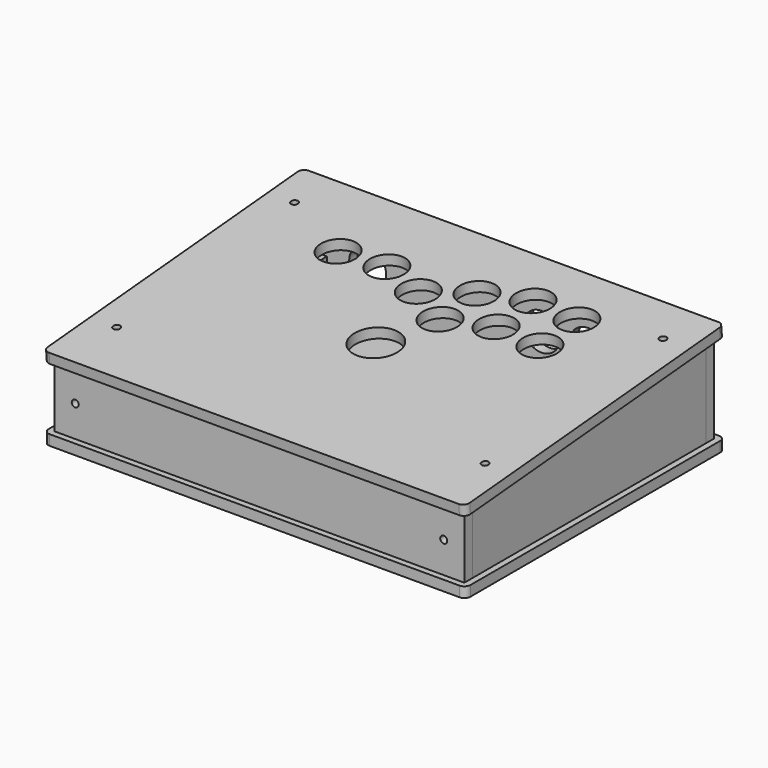
from build123d import *

# Parameters (mm, degrees)
F0_W      = 12.5984
F0_H      = 4.572
F0_W_2    = 3.048
F0_W_3    = 4.572
F0_H_2    = 12.5984
F0_H_3    = 3.048
F0_H_4    = 2.286
F0_W_4    = 2.286
F1_DEPTH  = 6.7056
F2_DEPTH  = 6.7056
F4_DEPTH  = 6.7056
F7_DEPTH  = 266.7
F8_R      = 2.286
F10_DEPTH = 6.7056
F9_R      = 2.286
F11_DEPTH = 6.7056
F12_W     = 266.7
F12_H     = 203.9761909888
F12_R     = 2.286
F12_R_2   = 15
F12_R_3   = 12
F12_W_2   = 6.7056
F12_H_2   = 190.5137623835
F13_DEPTH = 6.7056
F14_W     = 266.7
F14_H     = 203.2
F14_R     = 2.286
F14_W_2   = 6.7056
F14_H_2   = 189.7888
F15_DEPTH = 6.7056
F16_R     = 12
F16_R_2   = 1.6
F17_DEPTH = 6.7056


# Not quite as in the source:
# - a feature names something its author has since deleted; it is built from what else it names


with BuildPart() as f1:
    # F0 (on Right) → F1 (new body)
    with BuildSketch(Plane.YZ):
        Polygon((-94.8944, -2.286), (-94.8944, -20.32), (-69.4944, -20.32), (-69.4944, -7.7216), (-71.7804, -7.7216), (-71.7804, -4.6736), (-69.4944, -4.6736), (-69.4944, -1.6256), (-64.9224, -1.6256), (-64.9224, -4.6736), (-62.6364, -4.6736), (-62.6364, -7.7216), (-64.9224, -7.7216), (-64.9224, -20.32), (75.0824, -20.32), (75.0824, -7.7216), (72.7964, -7.7216), (72.7964, -4.6736), (75.0824, -4.6736), (75.0824, -1.6256), (79.6544, -1.6256), (79.6544, -4.6736), (81.9404, -4.6736), (81.9404, -7.7216), (79.6544, -7.7216), (79.6544, -20.32), (94.8944, -20.32), (94.8944, 6.6028482142), (82.296, 6.6028482142), (82.296, 4.3168482142), (79.248, 4.3168482142), (79.248, 6.6028482142), (76.2, 6.6028482142), (76.2, 11.1748482142), (79.248, 11.1748482142), (79.248, 13.4608482142), (82.296, 13.4608482142), (82.296, 11.1748482142), (94.8944, 11.1748482142), (94.8944, 37.5110324463), (79.7123928011, 36.1827789269), (80.8104157105, 23.6323196424), (83.0877167904, 23.8315576703), (83.3533674942, 20.7951562306), (81.0760664144, 20.5959182026), (81.3417171183, 17.5595167628), (76.7871149586, 17.161040707), (76.5214642547, 20.1974421468), (74.2441631749, 19.9982041189), (73.978512471, 23.0346055587), (76.2558135508, 23.2338435866), (75.1577906414, 35.784302871), (-65.0364525088, 23.5188959038), (-63.9384295994, 10.9684366193), (-61.6611285195, 11.1676746473), (-61.3954778156, 8.1312732075), (-63.6727788955, 7.9320351795), (-63.4071281916, 4.8956337398), (-67.9617303512, 4.4971576839), (-68.2273810551, 7.5335591237), (-70.504682135, 7.3343210958), (-70.7703328389, 10.3707225356), (-68.493031759, 10.5699605635), (-69.5910546685, 23.1204198479), (-94.8944, 20.9066639821), (-94.8944, 2.286), (-82.296, 2.286), (-82.296, 4.572), (-79.248, 4.572), (-79.248, 2.286), (-76.2, 2.286), (-76.2, -2.286), (-79.248, -2.286), (-79.248, -4.572), (-82.296, -4.572), (-82.296, -2.286), align=None)
        Polygon((79.7123928011, 36.1827789269), (75.1577906414, 35.784302871), (76.2558135508, 23.2338435866), (80.8104157105, 23.6323196424), align=None)
        Polygon((80.8104157105, 23.6323196424), (76.2558135508, 23.2338435866), (76.5214642547, 20.1974421468), (81.0760664144, 20.5959182026), align=None)
        Polygon((81.0760664144, 20.5959182026), (76.5214642547, 20.1974421468), (76.7871149586, 17.161040707), (81.3417171183, 17.5595167628), align=None)
        Polygon((-65.0364525088, 23.5188959038), (-69.5910546685, 23.1204198479), (-68.493031759, 10.5699605635), (-63.9384295994, 10.9684366193), align=None)
        Polygon((-63.9384295994, 10.9684366193), (-68.493031759, 10.5699605635), (-68.2273810551, 7.5335591237), (-63.6727788955, 7.9320351795), align=None)
        Polygon((-63.6727788955, 7.9320351795), (-68.2273810551, 7.5335591237), (-67.9617303512, 4.4971576839), (-63.4071281916, 4.8956337398), align=None)
        with Locations((-88.5952, 0)):
            Rectangle(F0_W, F0_H)
        with Locations((-80.772, 0)):
            Rectangle(F0_W_2, F0_H)
        with Locations((-77.724, 0)):
            Rectangle(F0_W_2, F0_H)
        with Locations((-67.2084, -14.0208)):
            Rectangle(F0_W_3, F0_H_2)
        with Locations((-67.2084, -6.1976)):
            Rectangle(F0_W_3, F0_H_3)
        with Locations((-67.2084, -3.1496)):
            Rectangle(F0_W_3, F0_H_3)
        with Locations((77.3684, -14.0208)):
            Rectangle(F0_W_3, F0_H_2)
        with Locations((77.3684, -6.1976)):
            Rectangle(F0_W_3, F0_H_3)
        with Locations((77.3684, -3.1496)):
            Rectangle(F0_W_3, F0_H_3)
        with Locations((88.5952, 8.8888482142)):
            Rectangle(F0_W, F0_H)
        with Locations((80.772, 8.8888482142)):
            Rectangle(F0_W_2, F0_H)
        with Locations((77.724, 8.8888482142)):
            Rectangle(F0_W_2, F0_H)
        Polygon((76.5214642547, 20.1974421468), (76.2558135508, 23.2338435866), (73.978512471, 23.0346055587), (74.2441631749, 19.9982041189), align=None)
        Polygon((83.0877167904, 23.8315576703), (80.8104157105, 23.6323196424), (81.0760664144, 20.5959182026), (83.3533674942, 20.7951562306), align=None)
        with Locations((80.772, 5.4598482142)):
            Rectangle(F0_W_2, F0_H_4)
        with Locations((80.772, 12.3178482142)):
            Rectangle(F0_W_2, F0_H_4)
        with Locations((80.7974, -6.1976)):
            Rectangle(F0_W_4, F0_H_3)
        with Locations((73.9394, -6.1976)):
            Rectangle(F0_W_4, F0_H_3)
        with Locations((-63.7794, -6.1976)):
            Rectangle(F0_W_4, F0_H_3)
        with Locations((-70.6374, -6.1976)):
            Rectangle(F0_W_4, F0_H_3)
        with Locations((-80.772, -3.429)):
            Rectangle(F0_W_2, F0_H_4)
        with Locations((-80.772, 3.429)):
            Rectangle(F0_W_2, F0_H_4)
        Polygon((-68.2273810551, 7.5335591237), (-68.493031759, 10.5699605635), (-70.7703328389, 10.3707225356), (-70.504682135, 7.3343210958), align=None)
        Polygon((-61.6611285195, 11.1676746473), (-63.9384295994, 10.9684366193), (-63.6727788955, 7.9320351795), (-61.3954778156, 8.1312732075), align=None)
    extrude(amount=-F1_DEPTH)


with BuildPart() as f2:
    # F0 (on Right) → F2 (new body)
    with BuildSketch(Plane.YZ):
        Polygon((-94.8944, -2.286), (-94.8944, -20.32), (-69.4944, -20.32), (-69.4944, -7.7216), (-71.7804, -7.7216), (-71.7804, -4.6736), (-69.4944, -4.6736), (-69.4944, -1.6256), (-64.9224, -1.6256), (-64.9224, -4.6736), (-62.6364, -4.6736), (-62.6364, -7.7216), (-64.9224, -7.7216), (-64.9224, -20.32), (75.0824, -20.32), (75.0824, -7.7216), (72.7964, -7.7216), (72.7964, -4.6736), (75.0824, -4.6736), (75.0824, -1.6256), (79.6544, -1.6256), (79.6544, -4.6736), (81.9404, -4.6736), (81.9404, -7.7216), (79.6544, -7.7216), (79.6544, -20.32), (94.8944, -20.32), (94.8944, 6.6028482142), (82.296, 6.6028482142), (82.296, 4.3168482142), (79.248, 4.3168482142), (79.248, 6.6028482142), (76.2, 6.6028482142), (76.2, 11.1748482142), (79.248, 11.1748482142), (79.248, 13.4608482142), (82.296, 13.4608482142), (82.296, 11.1748482142), (94.8944, 11.1748482142), (94.8944, 37.5110324463), (79.7123928011, 36.1827789269), (80.8104157105, 23.6323196424), (83.0877167904, 23.8315576703), (83.3533674942, 20.7951562306), (81.0760664144, 20.5959182026), (81.3417171183, 17.5595167628), (76.7871149586, 17.161040707), (76.5214642547, 20.1974421468), (74.2441631749, 19.9982041189), (73.978512471, 23.0346055587), (76.2558135508, 23.2338435866), (75.1577906414, 35.784302871), (-65.0364525088, 23.5188959038), (-63.9384295994, 10.9684366193), (-61.6611285195, 11.1676746473), (-61.3954778156, 8.1312732075), (-63.6727788955, 7.9320351795), (-63.4071281916, 4.8956337398), (-67.9617303512, 4.4971576839), (-68.2273810551, 7.5335591237), (-70.504682135, 7.3343210958), (-70.7703328389, 10.3707225356), (-68.493031759, 10.5699605635), (-69.5910546685, 23.1204198479), (-94.8944, 20.9066639821), (-94.8944, 2.286), (-82.296, 2.286), (-82.296, 4.572), (-79.248, 4.572), (-79.248, 2.286), (-76.2, 2.286), (-76.2, -2.286), (-79.248, -2.286), (-79.248, -4.572), (-82.296, -4.572), (-82.296, -2.286), align=None)
    extrude(amount=-F2_DEPTH)


with BuildPart() as f2_1:
    # F3: moved
    add(f2.part.moved(Location((-6.7056, 0, 0))))


with BuildPart() as f4:
    # F4 (new): a face of the model
    f4_faces = [f2_1.part.faces().sort_by_distance(p)[0] for p in [
        (-13.4112, 5.4126631939, 4.6812181823),
    ]]
    extrude(f4_faces, amount=F4_DEPTH)


with BuildPart() as f5_1:
    # F5: instance of F1
    add(f1.part.mirror(Plane.YZ))


with BuildPart() as f5_2:
    # F5: instance of F2
    add(f2_1.part.mirror(Plane.YZ))


with BuildPart() as f5_3:
    # F5: instance of F4
    add(f4.part.mirror(Plane.YZ))


with BuildPart() as f5_1_1:
    # F6: moved
    add(f5_1.part.moved(Location((-266.7, 0, 0))))


with BuildPart() as f5_2_1:
    # F6: moved
    add(f5_2.part.moved(Location((-266.7, 0, 0))))


with BuildPart() as f5_3_1:
    # F6: moved
    add(f5_3.part.moved(Location((-266.7, 0, 0))))


with BuildPart() as f7:
    # F0 (on Right) → F7 (new body, through all)
    with BuildSketch(Plane.YZ):
        Polygon((-101.6, 20.32), (-101.6, -20.32), (-94.8944, -20.32), (-94.8944, -2.286), (-94.8944, 2.286), (-94.8944, 20.9066639821), align=None)
    extrude(amount=-F7_DEPTH)

    # F8 (on face) → F10 (cut, through all)
    with BuildSketch(Plane(origin=(0, -94.8944, 0), x_dir=(-1, 0, 0), z_dir=(0, 1, 0))):
        with Locations((253.2888, 0)):
            Circle(F8_R)
        with Locations((13.4112, 0)):
            Circle(F8_R)
    extrude(amount=-F10_DEPTH, mode=Mode.SUBTRACT)


with BuildPart() as f7b:
    # F0 (on Right) → F7, piece 2 (new body, through all)
    with BuildSketch(Plane.YZ):
        Polygon((94.8944, 6.6028482142), (94.8944, -20.32), (101.6, -20.32), (101.6, 38.0976964285), (94.8944, 37.5110324463), (94.8944, 11.1748482142), align=None)
    extrude(amount=-F7_DEPTH)

    # F9 (on face) → F11 (cut, through all)
    with BuildSketch(Plane.XZ.offset(-94.8944)):
        with Locations((-253.2888, 8.8888482142)):
            Circle(F9_R)
        with Locations((-13.4112, 8.8888482142)):
            Circle(F9_R)
    extrude(amount=-F11_DEPTH, mode=Mode.SUBTRACT)

    # F16 (on face) → F17 (cut, through all)
    with BuildSketch(Plane(origin=(0, 101.6, 0), x_dir=(-1, 0, 0), z_dir=(0, 1, 0))):
        with Locations((46.5429987889, 8.8888482142)):
            Circle(F16_R)
        with Locations((76.7429987889, 8.8888482142)):
            Circle(F16_R)
        with Locations((220.1570012111, 8.8888482142)):
            Circle(F16_R)
        with Locations((106.9429987889, 8.8888482142)):
            Circle(F16_R)
        with Locations((210.6570012111, 20.8888482142)):
            Circle(F16_R_2)
        with Locations((229.6570012111, -3.1111517858)):
            Circle(F16_R_2)
    extrude(amount=-F17_DEPTH, mode=Mode.SUBTRACT)


with BuildPart() as f13:
    # F12 (on face) → F13 (new body)
    with BuildSketch(Plane(origin=(0, -2.5360316321, 28.9869741961), x_dir=(1, 0, 0), z_dir=(0, -0.0871557427, 0.9961946981))):
        with BuildLine():
            ThreePointArc((-266.7, 108.5338143553), (-269.5284271247, 107.3622414801), (-270.7, 104.5338143553))
            Line((-270.7, 104.5338143553), (-270.7, -99.4423766335))
            ThreePointArc((-270.7, -99.4423766335), (-269.5284271247, -102.2708037582), (-266.7, -103.4423766335))
            Line((-266.7, -103.4423766335), (0, -103.4423766335))
            ThreePointArc((0, -103.4423766335), (2.8284271247, -102.2708037582), (4, -99.4423766335))
            Line((4, -99.4423766335), (4, 104.5338143553))
            ThreePointArc((4, 104.5338143553), (2.8284271247, 107.3622414801), (0, 108.5338143553))
            Line((0, 108.5338143553), (-266.7, 108.5338143553))
        make_face()
        with Locations((-133.35, 2.5457188609)):
            Rectangle(F12_W, F12_H, mode=Mode.SUBTRACT)
        Polygon((0, 104.5338143553), (-266.7, 104.5338143553), (-266.7, -99.4423766335), (0, -99.4423766335), (0, -92.7111623309), (-6.7056, -92.7111623309), (-6.7056, 97.8026000527), (0, 97.8026000527), align=None)
        with Locations((-253.2888, -65.0251623309)):
            Circle(F12_R, mode=Mode.SUBTRACT)
        with Locations((-13.4112, -65.0251623309)):
            Circle(F12_R, mode=Mode.SUBTRACT)
        with Locations((-133.35, -3.8489602464)):
            Circle(F12_R_2, mode=Mode.SUBTRACT)
        with Locations((-205.0570012111, 55.3026000527)):
            Circle(F12_R_3, mode=Mode.SUBTRACT)
        with Locations((-146.4269835971, 47.3026000527)):
            Circle(F12_R_3, mode=Mode.SUBTRACT)
        with Locations((-253.2888, 80.2766000527)):
            Circle(F12_R, mode=Mode.SUBTRACT)
        with Locations((-174.9232991485, 57.3026000527)):
            Circle(F12_R_3, mode=Mode.SUBTRACT)
        with Locations((-120.2730164029, 32.2026000527)):
            Circle(F12_R_3, mode=Mode.SUBTRACT)
        with Locations((-91.7767008515, 42.2026000527)):
            Circle(F12_R_3, mode=Mode.SUBTRACT)
        with Locations((-61.6429987889, 40.2026000527)):
            Circle(F12_R_3, mode=Mode.SUBTRACT)
        with Locations((-120.2730164029, 62.4026000527)):
            Circle(F12_R_3, mode=Mode.SUBTRACT)
        with Locations((-91.7767008515, 72.4026000527)):
            Circle(F12_R_3, mode=Mode.SUBTRACT)
        with Locations((-61.6429987889, 70.4026000527)):
            Circle(F12_R_3, mode=Mode.SUBTRACT)
        with Locations((-13.4112, 80.2766000527)):
            Circle(F12_R, mode=Mode.SUBTRACT)
        with Locations((-3.3528, 2.5457188609)):
            Rectangle(F12_W_2, F12_H_2)
    extrude(amount=F13_DEPTH)


with BuildPart() as f15:
    # F14 (on face) → F15 (new body)
    with BuildSketch(Plane(origin=(0, 0, -20.32), x_dir=(1, 0, 0), z_dir=(0, 0, -1))):
        with BuildLine():
            ThreePointArc((-266.7, 105.6), (-269.5284271247, 104.4284271247), (-270.7, 101.6))
            Line((-270.7, 101.6), (-270.7, -101.6))
            ThreePointArc((-270.7, -101.6), (-269.5284271247, -104.4284271247), (-266.7, -105.6))
            Line((-266.7, -105.6), (0, -105.6))
            ThreePointArc((0, -105.6), (2.8284271247, -104.4284271247), (4, -101.6))
            Line((4, -101.6), (4, 101.6))
            ThreePointArc((4, 101.6), (2.8284271247, 104.4284271247), (0, 105.6))
            Line((0, 105.6), (-266.7, 105.6))
        make_face()
        with Locations((-133.35, 0)):
            Rectangle(F14_W, F14_H, mode=Mode.SUBTRACT)
        Polygon((0, 94.8944), (0, 101.6), (-266.7, 101.6), (-266.7, -101.6), (0, -101.6), (0, -94.8944), (-6.7056, -94.8944), (-6.7056, 94.8944), align=None)
        with Locations((-253.2888, -77.3684)):
            Circle(F14_R, mode=Mode.SUBTRACT)
        with Locations((-13.4112, -77.3684)):
            Circle(F14_R, mode=Mode.SUBTRACT)
        with Locations((-253.2888, 67.2084)):
            Circle(F14_R, mode=Mode.SUBTRACT)
        with Locations((-13.4112, 67.2084)):
            Circle(F14_R, mode=Mode.SUBTRACT)
        with Locations((-3.3528, 0)):
            Rectangle(F14_W_2, F14_H_2)
    extrude(amount=F15_DEPTH)


solid = Compound([f1.part, f2_1.part, f4.part, f5_1_1.part, f5_2_1.part, f5_3_1.part, f7.part, f7b.part, f13.part, f15.part])
